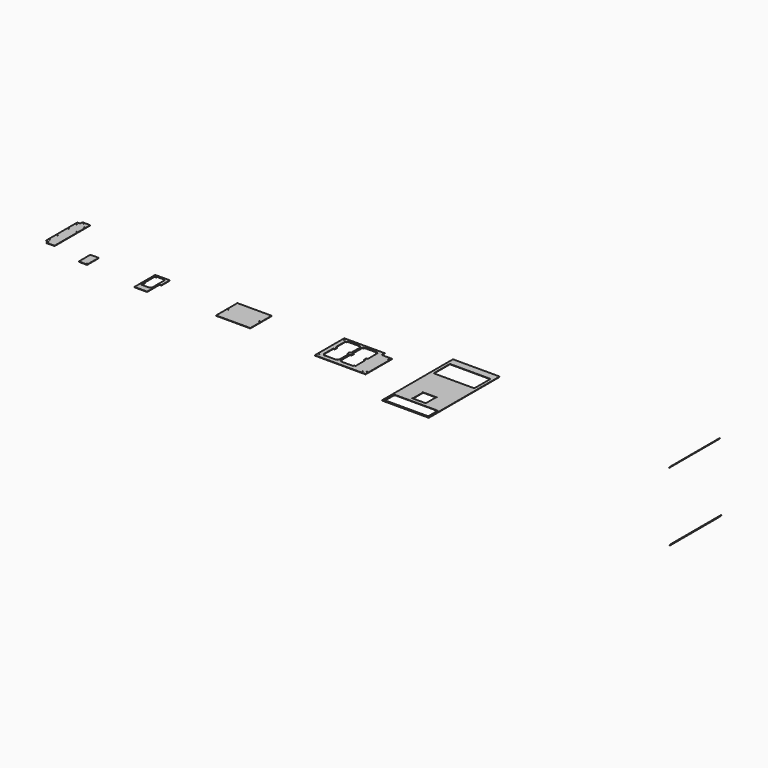
from build123d import *

# Parameters (mm, degrees)
F0_R      = 1.65
F1_DEPTH  = 3
F2_R      = 2.6
F2_R_2    = 1.65
F2_R_3    = 2.2
F3_DEPTH  = 3
F4_R      = 4
F5_D      = 5.25
F6_W      = 270
F6_H      = 210
F6_R      = 2.2
F7_DEPTH  = 3
F8_R      = 1.65
F9_DEPTH  = 3
F11_R     = 2.2
F12_DEPTH = 3
F14_DEPTH = 490
F15_R     = 1.7
F16_DEPTH = 25
F18_DEPTH = 490
F19_R     = 1.7
F20_DEPTH = 25
F21_R     = 2.1
F21_R_2   = 2.2
F22_DEPTH = 3


# Not quite as in the source:
# - ends of sketch curves that miss each other by under 0.0002 mm in the source are joined
# - a feature of the source that left no trace in its solid (it failed there, or was rolled back) is left out
# - a feature names something its author has since deleted; it is built from what else it names


with BuildPart() as f1:
    # F0 (on Top) → F1 (new body)
    with BuildSketch(Plane.XY):
        Polygon((-184, 349), (-184, -349), (-170, -349), (170, -349), (184, -349), (184, 349), align=None)
        with Locations((-169, -344.0016414119)):
            Circle(F0_R, mode=Mode.SUBTRACT)
        with Locations((-169.0367627935, -239.0016478477)):
            Circle(F0_R, mode=Mode.SUBTRACT)
        with Locations((-64, -344.0016414119)):
            Circle(F0_R, mode=Mode.SUBTRACT)
        with Locations((-50, -344.0016414119)):
            Circle(F0_R, mode=Mode.SUBTRACT)
        with Locations((-64.0367885365, -238.9281222651)):
            Circle(F0_R, mode=Mode.SUBTRACT)
        with Locations((-50.0367919688, -238.9183188541)):
            Circle(F0_R, mode=Mode.SUBTRACT)
        with Locations((-54.9631822882, -213.8447932715)):
            Circle(F0_R, mode=Mode.SUBTRACT)
        with Locations((-54.9631822882, -108.8447932715)):
            Circle(F0_R, mode=Mode.SUBTRACT)
        with BuildLine():
            ThreePointArc((-169.9980174903, -249.0019817241), (-168.5342523648, -245.4651668088), (-164.998017883, -244))
            Line((-164.998017883, -244), (0, -244))
            Line((0, -244), (165.1160954498, -244))
            ThreePointArc((165.1160954498, -244), (168.6098602912, -245.4231847639), (170.1147159762, -248.8825571067))
            Line((170.1147159762, -248.8825571067), (172.1117961468, -333.8825571067))
            ThreePointArc((172.1117961468, -333.8825571067), (170.6899908565, -337.4937648414), (167.1131756204, -339))
            Line((167.1131756204, -339), (-164.96432857, -339))
            ThreePointArc((-164.96432857, -339), (-168.4991617612, -337.5362344818), (-169.9643281773, -334.0019817241))
            Line((-169.9643281773, -334.0019817241), (-169.9980174903, -249.0019817241))
        make_face(mode=Mode.SUBTRACT)
        with Locations((55, -344.0016414119)):
            Circle(F0_R, mode=Mode.SUBTRACT)
        with Locations((69, -344.0016414119)):
            Circle(F0_R, mode=Mode.SUBTRACT)
        with Locations((54.9631822882, -238.8447932715)):
            Circle(F0_R, mode=Mode.SUBTRACT)
        with Locations((68.9631788559, -238.8349898605)):
            Circle(F0_R, mode=Mode.SUBTRACT)
        with Locations((54.9631822882, -213.8447932715)):
            Circle(F0_R, mode=Mode.SUBTRACT)
        with Locations((174, -344.0016414119)):
            Circle(F0_R, mode=Mode.SUBTRACT)
        with Locations((173.9631531129, -238.761464278)):
            Circle(F0_R, mode=Mode.SUBTRACT)
        with BuildLine():
            Line((46.5, -212.8447932715), (-46.5, -212.8447932715))
            ThreePointArc((-46.5, -212.8447932715), (-50.0355339059, -211.3803271775), (-51.5, -207.8447932715))
            Line((-51.5, -207.8447932715), (-51.5, -114.8447932715))
            ThreePointArc((-51.5, -114.8447932715), (-50.0355339059, -111.3092593656), (-46.5, -109.8447932715))
            Line((-46.5, -109.8447932715), (46.5, -109.8447932715))
            ThreePointArc((46.5, -109.8447932715), (50.0355339059, -111.3092593656), (51.5, -114.8447932715))
            Line((51.5, -114.8447932715), (51.5, -207.8447932715))
            ThreePointArc((51.5, -207.8447932715), (50.0355339059, -211.3803271775), (46.5, -212.8447932715))
        make_face(mode=Mode.SUBTRACT)
        with Locations((54.9631822882, -108.8447932715)):
            Circle(F0_R, mode=Mode.SUBTRACT)
        with BuildLine():
            Line((-155, 289), (155, 289))
            ThreePointArc((155, 289), (158.5355339059, 287.5355339059), (160, 284))
            Line((160, 284), (160, 134))
            ThreePointArc((160, 134), (158.5355339059, 130.4644660941), (155, 129))
            Line((155, 129), (-155, 129))
            ThreePointArc((-155, 129), (-158.5355339059, 130.4644660941), (-160, 134))
            Line((-160, 134), (-160, 284))
            ThreePointArc((-160, 284), (-158.5355339059, 287.5355339059), (-155, 289))
        make_face(mode=Mode.SUBTRACT)
    extrude(amount=F1_DEPTH)


with BuildPart() as f3:
    # F2 (on Top) → F3 (new body)
    with BuildSketch(Plane.XY):
        Polygon((-881.397524765, 150), (-881.397524765, -140), (-759.3974132538, -140), (-701.397524765, -140), (-579.3974132538, -140.000000596), (-481.397524765, -140.000000596), (-481.397524765, 119.999999404), (-561.397524765, 119.999999404), (-561.397524765, 149.9999993642), align=None)
        with Locations((-869.397524765, -111.5)):
            Circle(F2_R, mode=Mode.SUBTRACT)
        with Locations((-840.8975224495, -99.5)):
            Circle(F2_R_2, mode=Mode.SUBTRACT)
        with Locations((-735.8975224495, -99.5)):
            Circle(F2_R_2, mode=Mode.SUBTRACT)
        with Locations((-708.8974109383, -99.500000596)):
            Circle(F2_R_2, mode=Mode.SUBTRACT)
        with Locations((-603.8974109383, -99.500000596)):
            Circle(F2_R_2, mode=Mode.SUBTRACT)
        with Locations((-577.397524765, -134.000000596)):
            Circle(F2_R_3, mode=Mode.SUBTRACT)
        with Locations((-577.397524765, -124.000000596)):
            Circle(F2_R_3, mode=Mode.SUBTRACT)
        with Locations((-517.397524765, -134.000000596)):
            Circle(F2_R_3, mode=Mode.SUBTRACT)
        with Locations((-517.397524765, -124.000000596)):
            Circle(F2_R_3, mode=Mode.SUBTRACT)
        with Locations((-493.397524765, -112.0000007709)):
            Circle(F2_R, mode=Mode.SUBTRACT)
        with Locations((-869.397524765, 10)):
            Circle(F2_R, mode=Mode.SUBTRACT)
        with Locations((-840.8975224495, 5.5)):
            Circle(F2_R_2, mode=Mode.SUBTRACT)
        with Locations((-840.8975224495, 20.5)):
            Circle(F2_R_2, mode=Mode.SUBTRACT)
        Polygon((-837.3975377769, 121.0000020862), (-837.3975377769, 130.0000020862), (-739.3975377769, 130.0000020862), (-739.3975377769, 121.0000020862), (-737.3975377769, 121.0000020862), (-728.3975377769, 121.0000020862), (-728.3975224495, 25), (-730.3975224495, 25), (-739.3975224495, 25), (-739.3975224495, 10), (-739.3975224495, 1), (-730.3975224495, 1), (-728.3975224495, 1), (-728.3975224495, -95), (-730.3975224495, -95), (-739.3975224495, -95), (-739.3975224495, -104), (-837.3975224495, -104), (-837.3975224495, -95), (-846.3975224495, -95), (-848.3975224495, -95), (-848.3975224495, 1), (-846.3975224495, 1), (-837.3975224495, 1), (-837.3975224495, 10), (-837.3975224495, 25), (-846.3975224495, 25), (-848.3975224495, 25), (-848.397537777, 121.0000020862), (-839.397537777, 121.0000020862), align=None, mode=Mode.SUBTRACT)
        with Locations((-735.8975224495, 5.5)):
            Circle(F2_R_2, mode=Mode.SUBTRACT)
        with Locations((-735.8975224495, 20.5)):
            Circle(F2_R_2, mode=Mode.SUBTRACT)
        with Locations((-708.8974109383, 5.499999404)):
            Circle(F2_R_2, mode=Mode.SUBTRACT)
        with Locations((-708.8974109383, 20.499999404)):
            Circle(F2_R_2, mode=Mode.SUBTRACT)
        with Locations((-840.8975377769, 125.5000020862)):
            Circle(F2_R_2, mode=Mode.SUBTRACT)
        with Locations((-869.397524765, 132)):
            Circle(F2_R, mode=Mode.SUBTRACT)
        with Locations((-735.8975377769, 125.5000020862)):
            Circle(F2_R_2, mode=Mode.SUBTRACT)
        with Locations((-708.8974262657, 125.5000014901)):
            Circle(F2_R_2, mode=Mode.SUBTRACT)
        Polygon((-705.3974262657, 121.0000014901), (-705.3974262657, 130.0000014901), (-607.3974262657, 130.0000014901), (-607.3974262657, 121.0000014901), (-605.3974262657, 121.0000014901), (-596.3974262657, 121.0000014901), (-596.3974109382, 24.999999404), (-598.3974109382, 24.999999404), (-607.3974109383, 24.999999404), (-607.3974109383, 9.999999404), (-607.3974109383, 0.999999404), (-598.3974109383, 0.999999404), (-596.3974109382, 0.999999404), (-596.3974109383, -95.000000596), (-598.3974109383, -95.000000596), (-607.3974109383, -95.000000596), (-607.3974109383, -104.000000596), (-705.3974109383, -104.000000596), (-705.3974109383, -95.000000596), (-714.3974109383, -95.000000596), (-716.3974109383, -95.000000596), (-716.3974109383, 0.999999404), (-714.3974109383, 0.999999404), (-705.3974109383, 0.999999404), (-705.3974109383, 9.999999404), (-705.3974109383, 24.999999404), (-714.3974109383, 24.999999404), (-716.3974109383, 24.999999404), (-716.3974262657, 121.0000014901), (-707.3974262657, 121.0000014901), align=None, mode=Mode.SUBTRACT)
        with Locations((-603.8974109383, 5.499999404)):
            Circle(F2_R_2, mode=Mode.SUBTRACT)
        with Locations((-603.8974109383, 20.499999404)):
            Circle(F2_R_2, mode=Mode.SUBTRACT)
        with Locations((-493.3975247054, 29.9999992291)):
            Circle(F2_R, mode=Mode.SUBTRACT)
        with Locations((-603.8974262657, 125.5000014901)):
            Circle(F2_R_2, mode=Mode.SUBTRACT)
        with Locations((-493.3975298405, 99.9999992291)):
            Circle(F2_R, mode=Mode.SUBTRACT)
    extrude(amount=F3_DEPTH)

    # F4
    f4_edges = [f3.edges().sort_by_distance(p)[0] for p in [
        (-837.397522, 1, 1.5),
        (-837.397522, 25, 1.5),
        (-739.397522, 25, 1.5),
        (-739.397522, 1, 1.5),
        (-837.397522, -95, 1.5),
        (-739.397522, -95, 1.5),
        (-837.397538, 121.000002, 1.5),
        (-837.397538, 130.000002, 1.5),
        (-739.397538, 130.000002, 1.5),
        (-739.397538, 121.000002, 1.5),
        (-728.397538, 121.000002, 1.5),
        (-848.397538, 121.000002, 1.5),
    ]]
    fillet(f4_edges, radius=F4_R)

    # F5 (through all)
    with Locations(Plane(origin=(0, 0, 0), x_dir=(1, 0, 0), z_dir=(0, 0, -1))):
        with Locations((-869.397524765, -10), (-869.397524765, -132), (-493.3975247054, -29.9999992291), (-493.397524765, 112.0000007709)):
            Hole(F5_D / 2)


with BuildPart() as f7:
    # F6 (on Top) → F7 (new body)
    with BuildSketch(Plane.XY):
        with Locations((-1552.4095505809, 0)):
            Rectangle(F6_W, F6_H)
        with Locations((-1675.4095505809, 0)):
            Circle(F6_R, mode=Mode.SUBTRACT)
        with Locations((-1429.4095505809, 0)):
            Circle(F6_R, mode=Mode.SUBTRACT)
    extrude(amount=F7_DEPTH)


with BuildPart() as f9:
    # F8 (on Top) → F9 (new body)
    with BuildSketch(Plane.XY):
        with BuildLine():
            Line((-2316.8811880809, 82.5), (-2316.8811880809, -100))
            Line((-2316.8811880809, -100), (-2316.8811880809, -122.5))
            Line((-2316.8811880809, -122.5), (-2216.8811880809, -122.5))
            Line((-2216.8811880809, -122.5), (-2216.8811880809, -100))
            Line((-2216.8811880809, -100), (-2216.8811880809, -5))
            ThreePointArc((-2216.8811880809, -5), (-2215.4167219868, -1.4644660941), (-2211.8811880809, 0))
            Line((-2211.8811880809, 0), (-2206.8811880809, 0))
            ThreePointArc((-2206.8811880809, 0), (-2203.3456541749, 1.4644660941), (-2201.8811880809, 5))
            Line((-2201.8811880809, 5), (-2201.8811880809, 77.5))
            ThreePointArc((-2201.8811880809, 77.5), (-2203.3456541749, 81.0355339059), (-2206.8811880809, 82.5))
            Line((-2206.8811880809, 82.5), (-2216.8811880809, 82.5))
            Line((-2216.8811880809, 82.5), (-2316.8811880809, 82.5))
        make_face()
        with Locations((-2301.8811880809, -45)):
            Circle(F8_R, mode=Mode.SUBTRACT)
        with Locations((-2232.8811880809, -68.5)):
            Circle(F8_R, mode=Mode.SUBTRACT)
        with BuildLine():
            Line((-2237.5311880809, -72.5), (-2306.8811880809, -72.5))
            Line((-2306.8811880809, -72.5), (-2306.8811880809, -49.65))
            Line((-2306.8811880809, -49.65), (-2301.8811880809, -49.65))
            ThreePointArc((-2301.8811880809, -49.65), (-2297.2311880809, -45), (-2301.8811880809, -40.35))
            Line((-2301.8811880809, -40.35), (-2306.8811880809, -40.35))
            Line((-2306.8811880809, -40.35), (-2306.8811880809, 72.5))
            Line((-2306.8811880809, 72.5), (-2301.0311880809, 72.5))
            Line((-2301.0311880809, 72.5), (-2301.0311880809, 68.5))
            ThreePointArc((-2301.0311880809, 68.5), (-2296.3811880809, 63.85), (-2291.7311880809, 68.5))
            Line((-2291.7311880809, 68.5), (-2291.7311880809, 72.5))
            Line((-2291.7311880809, 72.5), (-2237.5311880809, 72.5))
            Line((-2237.5311880809, 72.5), (-2237.5311880809, 68.5))
            ThreePointArc((-2237.5311880809, 68.5), (-2236.1692346134, 65.2119534675), (-2232.8811880809, 63.85))
            Line((-2232.8811880809, 63.85), (-2226.8811880809, 63.85))
            Line((-2226.8811880809, 63.85), (-2226.8811880809, -63.85))
            Line((-2226.8811880809, -63.85), (-2232.8811880809, -63.85))
            ThreePointArc((-2232.8811880809, -63.85), (-2236.1692346134, -65.2119534675), (-2237.5311880809, -68.5))
            Line((-2237.5311880809, -68.5), (-2237.5311880809, -72.5))
        make_face(mode=Mode.SUBTRACT)
        with Locations((-2296.3811880809, 68.5)):
            Circle(F8_R, mode=Mode.SUBTRACT)
        with Locations((-2232.8811880809, 68.5)):
            Circle(F8_R, mode=Mode.SUBTRACT)
    extrude(amount=F9_DEPTH)


with BuildPart() as f12:
    # F11 (on Top) → F12 (new body)
    with BuildSketch(Plane.XY):
        with BuildLine():
            ThreePointArc((-2796.4271564484, -66.3103261323), (-2794.9626903543, -69.8458600382), (-2791.4271564484, -71.3103261323))
            Line((-2791.4271564484, -71.3103261323), (-2735.4271564484, -71.3103261323))
            ThreePointArc((-2735.4271564484, -71.3103261323), (-2731.8916225424, -69.8458600382), (-2730.4271564484, -66.3103261323))
            Line((-2730.4271564484, -66.3103261323), (-2730.4271564484, -45.3103261323))
            Line((-2730.4271564484, -45.3103261323), (-2730.4271564484, 16.6896738677))
            Line((-2730.4271564484, 16.6896738677), (-2730.4271564484, 37.6896738677))
            ThreePointArc((-2730.4271564484, 37.6896738677), (-2731.8916225424, 41.2252077737), (-2735.4271564484, 42.6896738677))
            Line((-2735.4271564484, 42.6896738677), (-2791.4271564484, 42.6896738677))
            ThreePointArc((-2791.4271564484, 42.6896738677), (-2794.9626903543, 41.2252077737), (-2796.4271564484, 37.6896738677))
            Line((-2796.4271564484, 37.6896738677), (-2796.4271564484, 16.6896738677))
            Line((-2796.4271564484, 16.6896738677), (-2796.4271564484, -45.3103261323))
            Line((-2796.4271564484, -45.3103261323), (-2796.4271564484, -66.3103261323))
        make_face()
        with Locations((-2789.4271564484, -64.3103261323)):
            Circle(F11_R, mode=Mode.SUBTRACT)
        with Locations((-2737.4271564484, -64.3103261323)):
            Circle(F11_R, mode=Mode.SUBTRACT)
        with Locations((-2789.4271564484, 35.6896738677)):
            Circle(F11_R, mode=Mode.SUBTRACT)
        with Locations((-2737.4271564484, 35.6896738677)):
            Circle(F11_R, mode=Mode.SUBTRACT)
    extrude(amount=F12_DEPTH)


with BuildPart() as f14:
    # F13 (on Front) → F14 (new body)
    with BuildSketch(Plane.XZ):
        Polygon((552.1922356603, -155.6886577127), (535.1922356603, -172.6886577127), (535.1922356603, -176.9312983998), (556.4348763474, -155.6886577127), align=None)
    extrude(amount=F14_DEPTH)

    # F15 (on face) → F16 (cut)
    with BuildSketch(Plane(origin=(356.06176703, 0, -356.06176703), x_dir=(0.7071067812, 0, 0.7071067812), z_dir=(0.7071067812, 0, -0.7071067812))):
        with Locations((268.3495534513, 3)):
            Circle(F15_R)
        with Locations((268.3495534513, 487)):
            Circle(F15_R)
    extrude(amount=-F16_DEPTH, mode=Mode.SUBTRACT)


with BuildPart() as f18:
    # F17 (on Front) → F18 (new body)
    with BuildSketch(Plane.XZ):
        Polygon((533.4103107452, 367.4547954072), (533.4103107452, 363.21215472), (541.8955921195, 371.6974360943), (537.6529514324, 371.6974360943), align=None)
    extrude(amount=F18_DEPTH)

    # F19 (on face) → F20 (cut)
    with BuildSketch(Plane(origin=(85.0990780126, 0, -85.0990780126), x_dir=(0, 1, 0), z_dir=(0.7071067812, 0, -0.7071067812))):
        with Locations((-3, 640.0078254947)):
            Circle(F19_R)
        with Locations((-487, 640.0078254947)):
            Circle(F19_R)
    extrude(amount=-F20_DEPTH, mode=Mode.SUBTRACT)


with BuildPart() as f22:
    # F21 (on Top) → F22 (new body)
    with BuildSketch(Plane.XY):
        with BuildLine():
            Line((-3105.6934249817, -1), (-3043.6934249817, 0))
            Line((-3043.6934249817, 0), (-3043.6934249817, 350))
            Line((-3043.6934249817, 350), (-3105.6934249817, 351))
            Line((-3105.6934249817, 351), (-3105.6934249817, 334))
            ThreePointArc((-3105.6934249817, 334), (-3105.6906908182, 333.8373358999), (-3105.6934249817, 333.6746717998))
            ThreePointArc((-3105.6934249817, 333.6746717998), (-3107.2252687521, 330.301801994), (-3110.6934249817, 329))
            Line((-3110.6934249817, 329), (-3127.6934249817, 329))
            Line((-3127.6934249817, 329), (-3127.6934249817, 21))
            Line((-3127.6934249817, 21), (-3110.6934249817, 21))
            ThreePointArc((-3110.6934249817, 21), (-3107.2252687521, 19.698198006), (-3105.6934249817, 16.3253282002))
            ThreePointArc((-3105.6934249817, 16.3253282002), (-3105.6906908182, 16.1626641001), (-3105.6934249817, 16))
            Line((-3105.6934249817, 16), (-3105.6934249817, -1))
        make_face()
        with Locations((-3116.5934249817, 43.431774044)):
            Circle(F21_R, mode=Mode.SUBTRACT)
        with Locations((-3116.5934249817, 120.031774044)):
            Circle(F21_R, mode=Mode.SUBTRACT)
        with Locations((-3085.6934249817, 11)):
            Circle(F21_R_2, mode=Mode.SUBTRACT)
        with Locations((-3054.7934249817, 43.431774044)):
            Circle(F21_R, mode=Mode.SUBTRACT)
        with Locations((-3054.7934249817, 120.031774044)):
            Circle(F21_R, mode=Mode.SUBTRACT)
        with Locations((-3116.5934249817, 229.968225956)):
            Circle(F21_R, mode=Mode.SUBTRACT)
        with Locations((-3116.5934249817, 306.568225956)):
            Circle(F21_R, mode=Mode.SUBTRACT)
        with Locations((-3054.7934249817, 229.968225956)):
            Circle(F21_R, mode=Mode.SUBTRACT)
        with Locations((-3085.6934249817, 339)):
            Circle(F21_R_2, mode=Mode.SUBTRACT)
        with Locations((-3054.7934249817, 306.568225956)):
            Circle(F21_R, mode=Mode.SUBTRACT)
    extrude(amount=F22_DEPTH)


with BuildPart() as f14_1:
    # F23: moved
    add(f14.part.moved(Location((1658, 0, 0))))


with BuildPart() as f18_1:
    # F23: moved
    add(f18.part.moved(Location((1658, 0, 0))))


solid = Compound([f1.part, f3.part, f7.part, f9.part, f12.part, f22.part, f14_1.part, f18_1.part])
